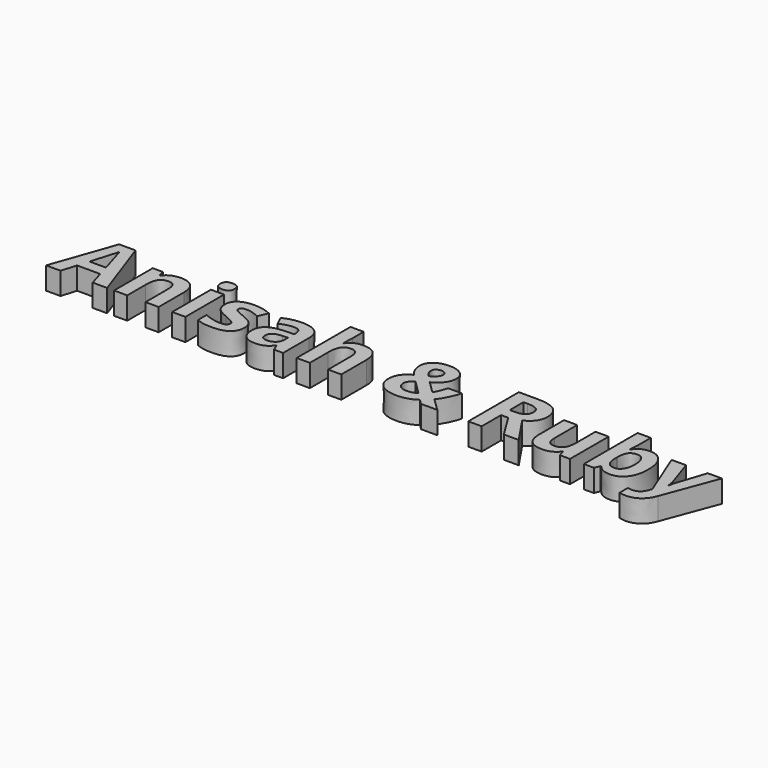
from build123d import *

# Parameters (mm, degrees)
F0_TEXT_SIZE = 63.4733380543
F1_DEPTH     = 16.002


# Not quite as in the source:
# - Text() gives the source's letters only with a copy of the font that has no kerning and outlines rounded to 1/6400 em; it was checked with that copy


with BuildPart() as f1:
    # F0 (on Top) → F1 (new body)
    with BuildSketch(Plane.XY):
        with Locations((0, 0)):
            Text('Anisah & Ruby', F0_TEXT_SIZE, font='Open Sans', font_style=FontStyle.BOLD, text_align=(TextAlign.LEFT, TextAlign.BOTTOM))
    extrude(amount=F1_DEPTH)


solid = f1.part
